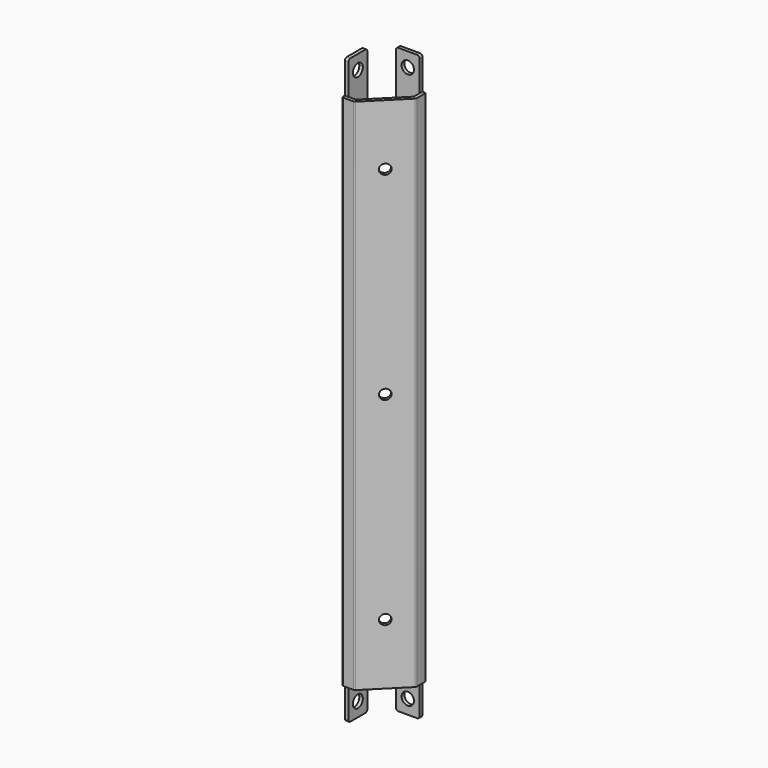
from build123d import *

# Parameters (mm, degrees)
F1_DEPTH = 247.5
F3_DEPTH = 28
F4_R     = 4.25
F5_DEPTH = 25
F6_R     = 5.25
F7_DEPTH = 25
F8_R     = 5.25
F9_DEPTH = 25
F10_R    = 2
F11_R    = 0.5
F12_R    = 1


# Not quite as in the source:
# - a pattern or mirror of a feature is missing from the dataset's text; its kind, count and spacing are read off the source's solid


with BuildPart() as f1:
    # F0 (on Top) → F1 (new body, symmetric)
    with BuildSketch(Plane.XY):
        Polygon((-19.75, 3.25), (-19.75, -19.75), (-9.25, -19.75), (19.75, 9.25), (19.75, 19.75), (-3.25, 19.75), (-3.25, 16.75), (16.75, 16.75), (16.75, 10.4926406871), (-10.4926406871, -16.75), (-16.75, -16.75), (-16.75, 3.25), align=None)
    extrude(amount=F1_DEPTH, both=True)

    # F2 (on face) → F3 (cut)
    with BuildSketch(Plane.XY.offset(247.5)):
        Polygon((-10.4926406871, -16.75), (-16.75, -16.75), (-19.75, -16.75), (-19.75, -19.75), (-9.25, -19.75), (19.75, 9.25), (19.75, 19.75), (16.75, 19.75), (16.75, 16.75), (16.75, 10.4926406871), align=None)
    f3 = extrude(amount=-F3_DEPTH, mode=Mode.SUBTRACT)

    # F3_copies: F3 across plane
    add(f3.mirror(Plane(origin=(0, 0, 0), x_dir=(-1, 0, 0), z_dir=(0, 0, -1))), mode=Mode.SUBTRACT)

    # F4 (on face) → F5 (cut)
    with BuildSketch(Plane(origin=(5.25, -5.25, 0), x_dir=(0.7071067812, 0.7071067812, 0), z_dir=(0.7071067812, -0.7071067812, 0))):
        with Locations((0, 168)):
            Circle(F4_R)
        with Locations((0, -168)):
            Circle(F4_R)
        Circle(F4_R)
    extrude(amount=-F5_DEPTH, mode=Mode.SUBTRACT)

    # F6 (on face) → F7 (cut)
    with BuildSketch(Plane.YZ.offset(-16.75)):
        with Locations((-6.75, 235.5)):
            Circle(F6_R)
        with Locations((-6.75, -235.5)):
            Circle(F6_R)
    extrude(amount=-F7_DEPTH, mode=Mode.SUBTRACT)

    # F8 (on face) → F9 (cut)
    with BuildSketch(Plane.XZ.offset(-16.75)):
        with Locations((6.75, 235.5)):
            Circle(F8_R)
        with Locations((6.75, -235.5)):
            Circle(F8_R)
    extrude(amount=-F9_DEPTH, mode=Mode.SUBTRACT)

    # F10
    f10_edges = [f1.edges().sort_by_distance(p)[0] for p in [
        (-9.25, -19.75, 0),
        (19.75, 9.25, 0),
        (-18.25, -16.75, 247.5),
        (-18.25, 3.25, 247.5),
        (-3.25, 18.25, 247.5),
        (16.75, 18.25, 247.5),
        (-18.25, 3.25, -247.5),
        (-3.25, 18.25, -247.5),
        (-18.25, -16.75, -247.5),
        (16.75, 18.25, -247.5),
    ]]
    fillet(f10_edges, radius=F10_R)

    # F11
    f11_edges = [f1.edges().sort_by_distance(p)[0] for p in [
        (-10.492641, -16.75, 0),
        (16.75, 10.492641, 0),
    ]]
    fillet(f11_edges, radius=F11_R)

    # F12
    f12_edges = [f1.edges().sort_by_distance(p)[0] for p in [
        (-19.75, -19.75, 0),
        (19.75, 19.75, 0),
    ]]
    fillet(f12_edges, radius=F12_R)


solid = f1.part
